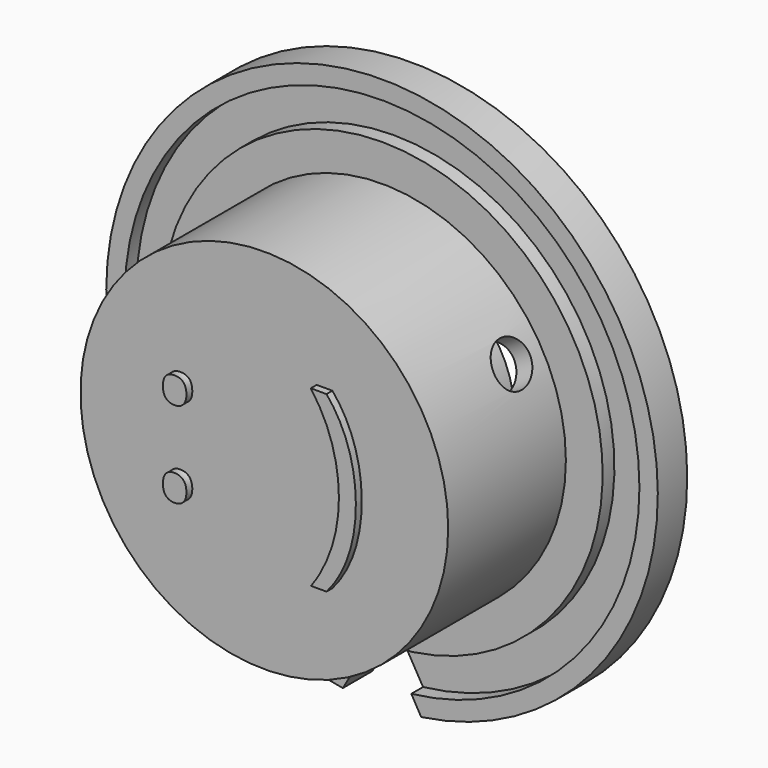
from build123d import *

# Parameters (mm, degrees)
F0_R          = 37.5
F1_DEPTH      = 5
F2_R          = 25
F3_DEPTH      = 20
F5_DEPTH      = 25
F6_R          = 10.25
F7_DEPTH      = 20
F8_R          = 22.5
F8_R_2        = 14
F9_DEPTH      = 20
F11_R         = 3
F12_DEPTH     = 25
F16_DEPTH     = 25
F17_TEXT_SIZE = 27.1109855973
F18_DEPTH     = 1
F20_DEPTH     = 2


# Not quite as in the source:
# - Text() gives the source's letters only with a copy of the font that has no kerning and outlines rounded to 1/6400 em; it was checked with that copy


with BuildPart() as f1:
    # F0 (on Front) → F1 (new body)
    with BuildSketch(Plane.XZ):
        Circle(F0_R)
    extrude(amount=F1_DEPTH)

    # F2 (on face) → F3 (join)
    with BuildSketch(Plane.XZ.offset(5)):
        Circle(F2_R)
    extrude(amount=F3_DEPTH)

    # F4 (on face) → F5 (cut)
    with BuildSketch(Plane.XZ.offset(5)):
        with BuildLine():
            ThreePointArc((-5.3323374343, -37.1189463413), (-2.672967658, -37.4046152754), (0, -37.5))
            ThreePointArc((0, -37.5), (2.672967658, -37.4046152754), (5.3323374343, -37.1189463413))
            Line((5.3323374343, -37.1189463413), (0, -27.883066982))
            Line((0, -27.883066982), (-5.3323374343, -37.1189463413))
        make_face()
    extrude(amount=-F5_DEPTH, mode=Mode.SUBTRACT)

    # F6 (on face) → F7 (cut)
    with BuildSketch(Plane(origin=(0, 0, 0), x_dir=(-1, 0, 0), z_dir=(0, 1, 0))):
        Circle(F6_R)
    extrude(amount=-F7_DEPTH, mode=Mode.SUBTRACT)

    # F8 (on face) → F9 (cut)
    with BuildSketch(Plane(origin=(0, 0, 0), x_dir=(-1, 0, 0), z_dir=(0, 1, 0))):
        Circle(F8_R)
        Circle(F8_R_2, mode=Mode.SUBTRACT)
    extrude(amount=-F9_DEPTH, mode=Mode.SUBTRACT)

    # F11 (on offset) → F12 (cut)
    with BuildSketch(Plane.XY.offset(-25)):
        with Locations((0, -10)):
            Circle(F11_R)
    extrude(amount=F12_DEPTH, mode=Mode.SUBTRACT)

    # F15 (on line) → F16 (cut)
    with BuildSketch(Plane(origin=(21.6506350946, 0, 12.5), x_dir=(0, 1, 0), z_dir=(0.8660254038, 0, 0.5))):
        with BuildLine():
            Line((-7, 0), (-13, 0))
            ThreePointArc((-13, 0), (-10, -3), (-7, 0))
        make_face()
        with BuildLine():
            ThreePointArc((-7, 0), (-10, 3), (-13, 0))
            Line((-13, 0), (-7, 0))
        make_face()
    extrude(amount=-F16_DEPTH, mode=Mode.SUBTRACT)

    # F17 (on face) → F18 (join)
    with BuildSketch(Plane.XZ.offset(25)):
        with Locations((-15, -8)):
            Text(':  )', F17_TEXT_SIZE, font='Open Sans', text_align=(TextAlign.LEFT, TextAlign.BOTTOM))
    extrude(amount=F18_DEPTH)

    # F19 (on face) → F20 (cut)
    with BuildSketch(Plane.XZ.offset(5)):
        with BuildLine():
            ThreePointArc((-1.2081606391, -29.9756625927), (-20.7816647652, 21.6361366604), (30, 0))
            ThreePointArc((30, 0), (21.6361366604, -20.7816647652), (1.2081606391, -29.9756625927))
            Line((1.2081606391, -29.9756625927), (3.9780195096, -34.7731988862))
            ThreePointArc((3.9780195096, -34.7731988862), (26.1173379466, -23.299885377), (35, 0))
            ThreePointArc((35, 0), (-23.299885377, 26.1173379466), (-3.9780195096, -34.7731988862))
            Line((-3.9780195096, -34.7731988862), (-1.2081606391, -29.9756625927))
        make_face()
    extrude(amount=-F20_DEPTH, mode=Mode.SUBTRACT)


solid = f1.part
